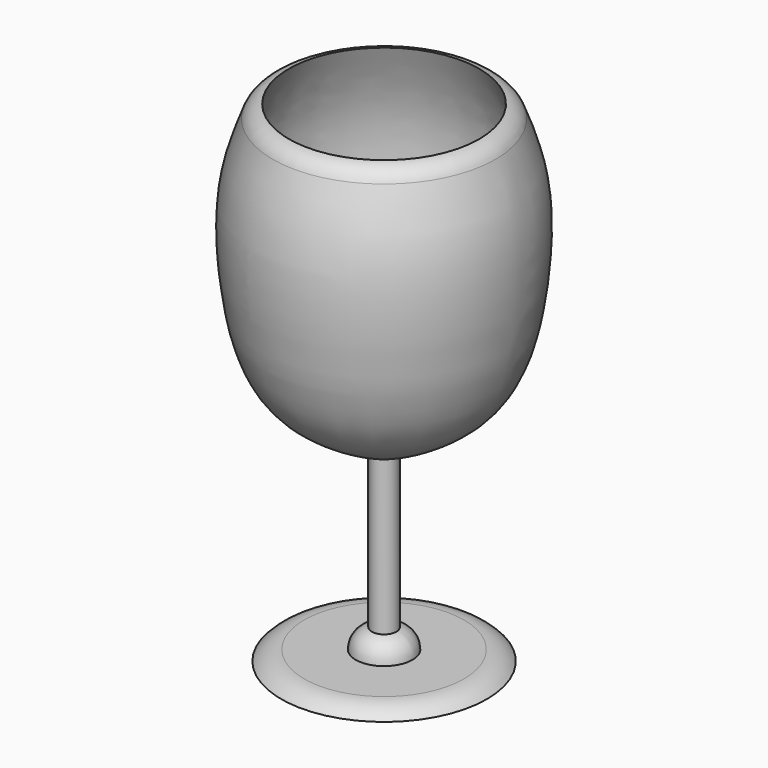
from build123d import *


# Not quite as in the source:
# - a fillet or chamfer that OpenCascade refuses, or shapes differently, is made with other operations: its cross-section is extruded or revolved along the edge and cut away or added
# - the dataset's text gives a spline's control points without its knots; the knots are read off the source's solid


with BuildPart() as f1:
    # F0 (on Front) → F1 (revolve)
    with BuildSketch(Plane.XZ):
        with BuildLine():
            Line((0, 47.7505947651), (0, 0))
            Line((0, 0), (25.4, 0))
            Line((25.4, 0), (25.4, 2.54))
            Line((25.4, 2.54), (6.9873421453, 2.54))
            Line((6.9873421453, 2.54), (6.9873421453, 7.3809963651))
            Line((6.9873421453, 7.3809963651), (3.0508127529, 7.3809963651))
            Line((3.0508127529, 7.3809963651), (3.0508127529, 45.4809963651))
            add(Edge.make_bspline(
                [(3.0508127529, 45.4809963651), (9.8461281639, 48.8954375707), (21.7228349186, 54.8631247901), (28.2240876429, 65.9165943611), (31.5127213678, 78.4358206865), (33.6784171743, 103.0849392109), (28.386283274, 115.9113566716), (25.8480589837, 122.0631897449)],
                knots=[0, 0, 0, 0, 0.2177295257, 0.3805430023, 0.5507700364, 0.7845393886, 1, 1, 1, 1], degree=3))
            Line((25.8480589837, 122.0631897449), (23.5000647508, 121.0944157349))
            add(Edge.make_bspline(
                [(1.9104079551, 47.7505947651), (3.8610263285, 48.7307217125), (7.7368881371, 50.6784180709), (12.2259767295, 53.1394673421), (15.4202565252, 55.1450698166), (17.2113496311, 56.4137046376), (18.4985579441, 57.4361542965), (19.3831690783, 58.2033768453), (20.1915430594, 58.9776879327), (21.1841928439, 60.0273218326), (22.2759624919, 61.3698248404), (23.392344712, 63.0381272524), (24.353200167, 64.7712061983), (25.0530786649, 66.2746693843), (25.5687607147, 67.5124472772), (26.0517126553, 68.761934225), (26.8207352465, 71.0094584469), (27.5553728133, 73.8128228874), (28.1157522153, 76.6310441845), (28.4178367466, 78.3658990039), (28.7101517328, 80.190879424), (29.0504794951, 82.6183883543), (29.5115503692, 86.7396383327), (29.8033217447, 91.1030083431), (29.8407350232, 95.4791342687), (29.7215088128, 98.7091824899), (29.4842699418, 101.3065910758), (29.202697145, 103.2994868111), (28.8607016819, 105.2540587373), (28.3291470633, 107.6283352293), (27.2887198112, 111.3164298649), (25.6928207945, 115.7785494719), (24.236343262, 119.3099152425), (23.5000647508, 121.0944157349)],
                knots=[4e-10, 4e-10, 4e-10, 4e-10, 0.0625000004, 0.1250000003, 0.1562500003, 0.1875000003, 0.2031250003, 0.2187500003, 0.2343750003, 0.2500000003, 0.2812500003, 0.3125000003, 0.3437500003, 0.3750000002, 0.3906250002, 0.4062500002, 0.4375000002, 0.5000000002, 0.5312500002, 0.5468750002, 0.5625000002, 0.5937500002, 0.6250000001, 0.6875000001, 0.7187500001, 0.7500000001, 0.7812500001, 0.7968750001, 0.8125000001, 0.8437500001, 0.875, 0.9375, 1, 1, 1, 1], degree=3))
            Line((1.9104079551, 47.7505947651), (0, 47.7505947651))
        make_face()
    revolve(axis=Axis((0, 0, 23.8752973825), (0, 0, -1)))

    # F2: fillet of radius 4.826 on 1 edges, made by hand

    # F2_s1 → F2_t2 (revolve, cut)
    with BuildSketch(Plane.XZ):
        with BuildLine():
            ThreePointArc((6.9873421453, 2.6376728427), (5.8750236847, 5.7196925415), (3.0508127529, 7.3809963651))
            Line((3.0508127529, 7.3809963651), (6.9873421453, 7.3809963651))
            Line((6.9873421453, 7.3809963651), (6.9873421453, 2.6376728427))
        make_face()
    revolve(axis=Axis((0, 0, 7.3809963651), (0, 0, -1)), mode=Mode.SUBTRACT)

    # F3: fillet of radius 7.62 on 1 edges, made by hand

    # F3_s1 → F3_t2 (revolve, cut)
    with BuildSketch(Plane.XZ):
        with BuildLine():
            ThreePointArc((19.7203873372, 2.54), (22.8312393105, 1.8760764803), (25.4, 0))
            Line((25.4, 0), (25.4, 2.54))
            Line((25.4, 2.54), (19.7203873372, 2.54))
        make_face()
    revolve(axis=Axis((0, 0, 2.54), (0, 0, -1)), mode=Mode.SUBTRACT)

    # F4: fillet of radius 5.08 on 1 edges, made by hand

    # F4_s1 → F4_t2 (revolve, cut)
    with BuildSketch(Plane.XZ):
        with BuildLine():
            ThreePointArc((23.5001194129, 121.0948119824), (25.9427148586, 120.0585616678), (27.5299870338, 117.93237864))
            Line((27.5299870338, 117.93237864), (28.0024132618, 118.1195048845))
            ThreePointArc((28.0024132618, 118.1195048845), (27.1665806291, 120.1928354079), (26.3177840752, 122.2569966352))
            Line((26.3177840752, 122.2569966352), (25.6542520935, 122.5329148365))
            ThreePointArc((25.6542520935, 122.5329148365), (24.4803481858, 122.048566289), (23.5695588788, 121.5981815612))
            Line((23.5695588788, 121.5981815612), (23.5001194129, 121.0948119824))
        make_face()
    revolve(axis=Axis((0, 0, 122.0631897449), (0, 0, -1)), mode=Mode.SUBTRACT)


solid = f1.part
